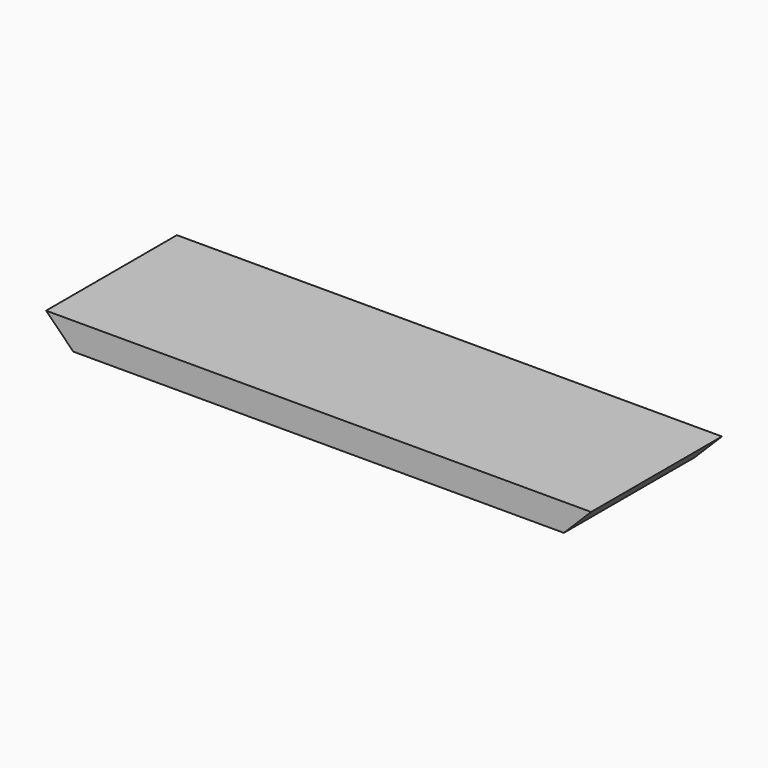
from build123d import *

# Parameters (mm, degrees)
F0_W     = 508
F0_H     = 25.4
F1_DEPTH = 152.4
F2_SIZE  = 25.39999


# Not quite as in the source:
# - a fillet or chamfer is up to 0.001 mm smaller than in the source, because OpenCascade refuses the exact size


with BuildPart() as f1:
    # F0 (on Front) → F1 (new body)
    with BuildSketch(Plane.XZ):
        Rectangle(F0_W, F0_H)
    extrude(amount=F1_DEPTH)

    # F2 (size 25.4 in the source; OpenCascade refuses exactly that, so slightly less here)
    f2_edges = [f1.edges().sort_by_distance(p)[0] for p in [
        (-254, -76.2, -12.7),
        (254, -76.2, -12.7),
    ]]
    chamfer(f2_edges, length=F2_SIZE)


solid = f1.part
